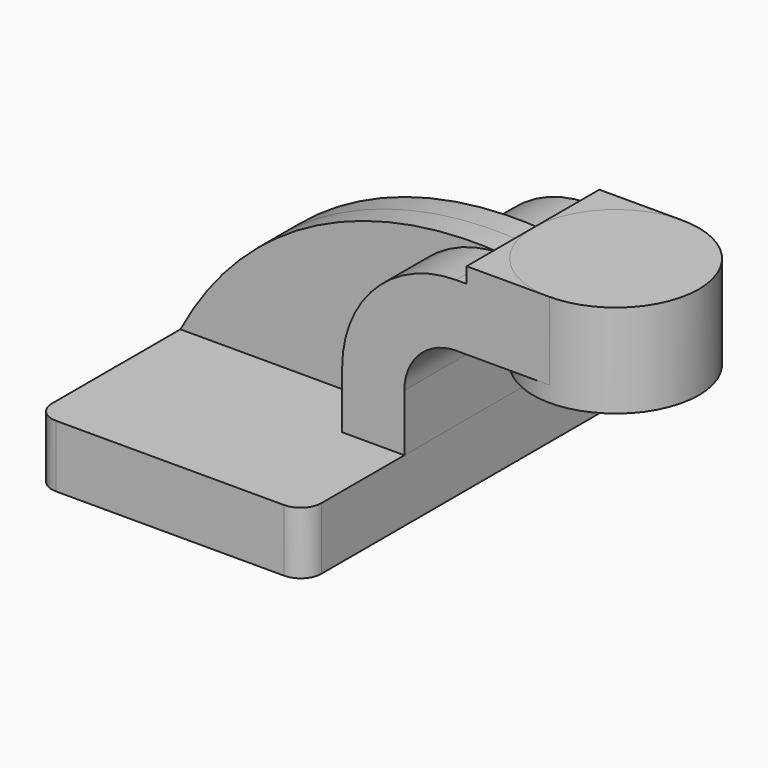
from build123d import *

# Parameters (mm, degrees)
F1_DEPTH = 63.5
F2_DEPTH = 25.4
F3_DEPTH = 7.9375
F5_R     = 6.35


# Not quite as in the source:
# - a feature names something its author has since deleted; it is built from what else it names


with BuildPart() as f1:
    # F0 (on Front) → F1 (new body, symmetric)
    with BuildSketch(Plane.XZ):
        Polygon((-41.275, 9.525), (-41.275, -9.525), (41.275, -9.525), (41.275, 9.525), (22.225, 9.525), align=None)
    extrude(amount=F1_DEPTH, both=True)

    # F5
    f5_edges = [f1.edges().sort_by_distance(p)[0] for p in [
        (41.275, -63.5, 0),
        (-41.275, -63.5, 0),
        (41.275, 63.5, 0),
        (-41.275, 63.5, 0),
    ]]
    fillet(f5_edges, radius=F5_R)


with BuildPart() as f2:
    # F0 (on Front) → F2 (new body, symmetric)
    with BuildSketch(Plane.XZ):
        with BuildLine():
            Line((22.225, 9.525), (41.275, 9.525))
            Line((41.275, 9.525), (41.275, 27.0002))
            ThreePointArc((41.275, 27.0002), (45.9246798487, 38.2255201513), (57.15, 42.8752))
            Line((57.15, 42.8752), (60.325, 42.8752))
            Line((60.325, 42.8752), (60.325, 61.9252))
            Line((60.325, 61.9252), (57.15, 61.9252))
            ThreePointArc((57.15, 61.9252), (32.4542956671, 51.6959043329), (22.225, 27.0002))
            Line((22.225, 27.0002), (22.225, 9.525))
        make_face()
        Polygon((60.325, 66.675), (60.325, 61.9252), (60.325, 42.8752), (85.725, 42.8752), (85.725, 66.675), align=None)
    extrude(amount=F2_DEPTH, both=True)


with BuildPart() as f3:
    # F0 (on Front) → F3 (new body, symmetric)
    with BuildSketch(Plane.XZ):
        with BuildLine():
            add(Edge.make_bspline(
                [(-41.275, 9.525), (-18.2747505605, 53.0267395079), (24.5660636574, 64.4110143185), (57.15, 61.9252)],
                knots=[0, 0, 0, 0, 111.5045361635, 111.5045361635, 111.5045361635, 111.5045361635], degree=3))
            Line((-41.275, 9.525), (22.225, 9.525))
            Line((22.225, 9.525), (22.225, 27.0002))
            ThreePointArc((22.225, 27.0002), (32.4542956671, 51.6959043329), (57.15, 61.9252))
        make_face()
    extrude(amount=F3_DEPTH, both=True)


with BuildPart() as f4:
    # F0 (on Front) → F4 (revolve)
    with BuildSketch(Plane.XZ):
        Polygon((85.725, 66.675), (85.725, 42.8752), (85.725, 38.1), (111.125, 38.1), (111.125, 66.675), align=None)
    revolve(axis=Axis((85.725, 0, 52.3875), (0, 0, 1)))


solid = Compound([f1.part, f2.part, f3.part, f4.part])
